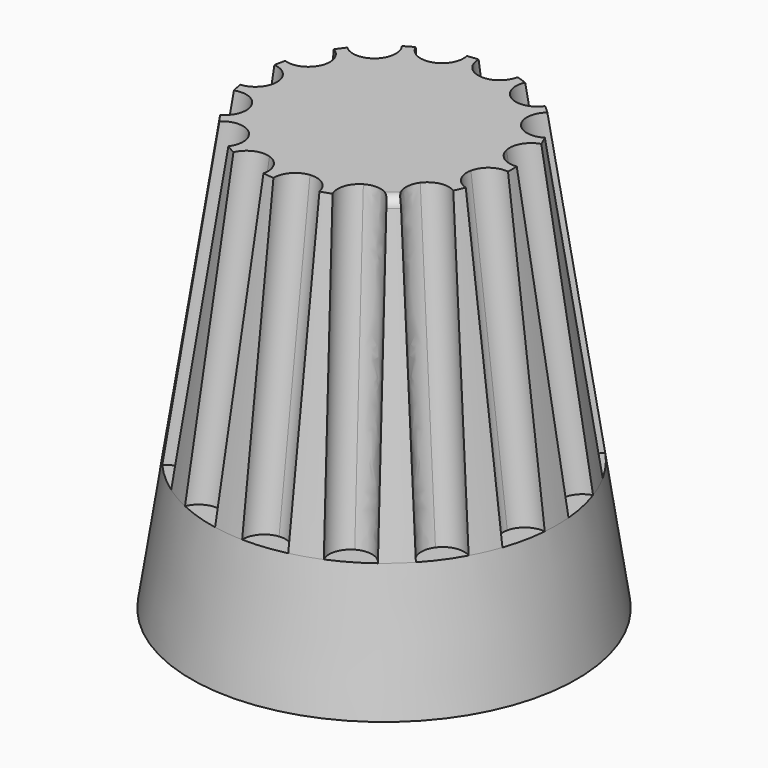
from build123d import *

# Parameters (mm, degrees)
F3_COPIES_COUNT = 15
F4_R            = 4
F5_DEPTH        = 16
F6_R            = 0.5
F7_R            = 1


# Not quite as in the source:
# - a pattern or mirror of a feature is missing from the dataset's text; its kind, count and spacing are read off the source's solid


with BuildPart() as f1:
    # F0 (on Front) → F1 (revolve)
    with BuildSketch(Plane.XZ):
        Polygon((-12.1391670853, 18.5), (-12.1391670853, 20), (-18.1391670853, 20), (-20.2312287555, 6.0529221986), (-21.1391670853, 0), (-19.655762556, -0.2225106794), (-16.8473859541, 18.5), align=None)
    revolve(axis=Axis((-12.1391670853, 0, -7.0133839902), (0, 0, -1)))

    # F3: sweep along a path in F0
    with BuildLine(Plane.XZ) as f3_path:
        Line((-18.1391670853, 20), (-20.2312287555, 6.0529221986))
    # F2 (on face) → F3 (sweep, cut)
    with BuildSketch(Plane.XY.offset(20)):
        with BuildLine():
            ThreePointArc((-18.055833752, -0.9965217286), (-18.1391670853, 0), (-18.055833752, 0.9965217286))
            ThreePointArc((-18.055833752, 0.9965217286), (-19.1391670853, 0), (-18.055833752, -0.9965217286))
        make_face()
        with BuildLine():
            ThreePointArc((-18.055833752, -0.9965217286), (-17.4031870131, -0.6770032004), (-17.1391670853, 0))
            ThreePointArc((-17.1391670853, 0), (-17.4031870131, 0.6770032004), (-18.055833752, 0.9965217286))
            ThreePointArc((-18.055833752, 0.9965217286), (-18.1391670853, 0), (-18.055833752, -0.9965217286))
        make_face()
    f3 = sweep(path=f3_path.line, mode=Mode.SUBTRACT)

    # F3_copies: F3 ×15 about axis
    f3_copies_axis = Axis((-12.139167, 0, 0), (0, 0, 1))
    for i in range(1, F3_COPIES_COUNT):
        add(f3.rotate(f3_copies_axis, i * 360 / F3_COPIES_COUNT), mode=Mode.SUBTRACT)

    # F4 (on face) → F5 (join)
    with BuildSketch(Plane(origin=(0, 0, 18.5), x_dir=(1, 0, 0), z_dir=(0, 0, -1))):
        with Locations((-12.1391670853, 0)):
            Circle(F4_R)
        with BuildLine():
            ThreePointArc((-13.7391670853, 2.5377155081), (-10.6900294107, 2.6267851073), (-9.1391670853, 0))
            ThreePointArc((-9.1391670853, 0), (-10.6900294107, -2.6267851073), (-13.7391670853, -2.5377155081))
            ThreePointArc((-13.7391670853, -2.5377155081), (-15.1391670853, 0), (-13.7391670853, 2.5377155081))
        make_face(mode=Mode.SUBTRACT)
    extrude(amount=F5_DEPTH)

    # F6
    f6_edges = [f1.edges().sort_by_distance(p)[0] for p in [
        (-8.124383, -4.458869, 20),
    ]]
    fillet(f6_edges, radius=F6_R)

    # F7
    f7_edges = [f1.edges().sort_by_distance(p)[0] for p in [
        (-4.622572, 0, -0.222511),
    ]]
    fillet(f7_edges, radius=F7_R)


solid = f1.part
